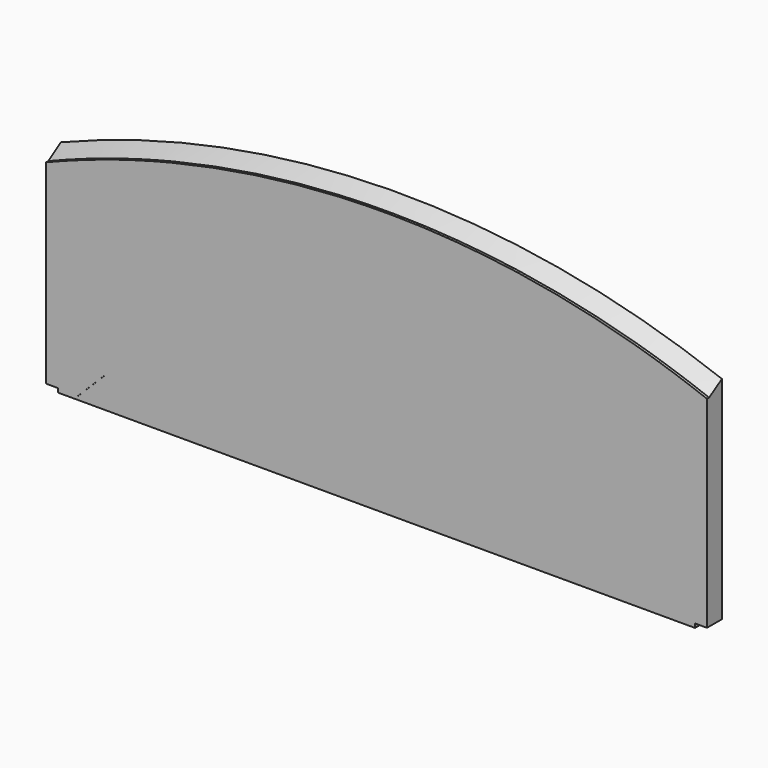
from build123d import *

# Parameters (mm, degrees)
F1_DEPTH    = 19.05
F2_T2_ANGLE = 47.80727079
F4_DEPTH    = 3.175


# Not quite as in the source:
# - a fillet or chamfer that OpenCascade refuses, or shapes differently, is made with other operations: its cross-section is extruded or revolved along the edge and cut away or added


with BuildPart() as f1:
    # F0 (on Front) → F1 (new body)
    with BuildSketch(Plane.XZ):
        with BuildLine():
            Line((-379.386894745, -118.26875), (379.4125, -118.26875))
            Line((379.4125, -118.26875), (379.4125, -113.50625))
            Line((379.4125, -113.50625), (393.7, -113.50625))
            Line((393.7, -113.50625), (393.7, 124.61875))
            ThreePointArc((393.7, 124.61875), (-0.5889314831, 196.0563533265), (-393.674394745, 118.26875))
            Line((-393.674394745, 118.26875), (-393.674394745, -113.50625))
            Line((-393.674394745, -113.50625), (-379.386894745, -113.50625))
            Line((-379.386894745, -113.50625), (-379.386894745, -118.26875))
        make_face()
        with BuildLine():
            ThreePointArc((-393.674394745, 118.26875), (-0.5889314831, 196.0563533265), (393.7, 124.61875))
            Line((393.7, 124.61875), (393.7, 138.90625))
            ThreePointArc((393.7, 138.90625), (-0.7824585401, 208.7544433839), (-393.7768174305, 130.96875))
            Line((-393.7768174305, 130.96875), (-393.674394745, 118.26875))
        make_face()
    extrude(amount=F1_DEPTH)

    # F2: chamfer of 19.558 x 11.43 on 1 edges, made by hand

    # F2_s1 → F2_t2 (revolve, cut)
    with BuildSketch(Plane(origin=(327.911656241, 0, -141.3984070605), x_dir=(0, 1, 0), z_dir=(0.9182658757, 0, -0.3959643691))):
        Polygon((0.508, 284.621375818), (-19.05, 273.191375818), (-19.05, 284.621375818), align=None)
    revolve(axis=Axis((10.1741912427, -19.05, -878.2512511865), (0, -1, 0)), revolution_arc=F2_T2_ANGLE, mode=Mode.SUBTRACT)

    # F3 (on face) → F4 (join)
    with BuildSketch(Plane.XZ.offset(19.05)):
        Polygon((71.1841804533, -118.26875), (178.9472539061, -118.26875), (218.205169263, -79.0108346431), (164.3236325366, -25.1292979167), (110.4420958102, -79.0108346431), align=None)
        Polygon((218.205169263, -79.0108346431), (178.9472539061, -118.26875), (257.4630846199, -118.26875), align=None)
        Polygon((393.7, -113.50625), (393.7, -38.9795184745), (379.8497794422, -25.1292979167), (325.9682427158, -79.0108346431), (286.710327359, -118.26875), (379.4125, -118.26875), (379.4125, -113.50625), align=None)
        Polygon((379.8497794422, -25.1292979167), (393.7, -38.9795184745), (393.7, -11.279077359), align=None)
        Polygon((218.205169263, -79.0108346431), (257.4630846199, -118.26875), (286.710327359, -118.26875), (325.9682427158, -79.0108346431), (272.0867059894, -25.1292979167), (218.205169263, 28.7522388097), (164.3236325366, -25.1292979167), align=None)
        Polygon((41.9369377142, -118.26875), (71.1841804533, -118.26875), (110.4420958102, -79.0108346431), (56.5605590837, -25.1292979167), (2.6790223573, 28.7522388097), (-51.2025143691, -25.1292979167), (2.6790223573, -79.0108346431), align=None)
        Polygon((-36.5788929995, -118.26875), (41.9369377142, -118.26875), (2.6790223573, -79.0108346431), align=None)
        Polygon((-144.3419664524, -118.26875), (-36.5788929995, -118.26875), (2.6790223573, -79.0108346431), (-51.2025143691, -25.1292979167), (-105.0840510955, -79.0108346431), align=None)
        Polygon((325.9682427158, -79.0108346431), (379.8497794422, -25.1292979167), (393.7, -11.279077359), (393.7, 68.7835549784), (379.8497794422, 82.6337755361), (325.9682427158, 28.7522388097), (272.0867059894, -25.1292979167), align=None)
        Polygon((110.4420958102, -79.0108346431), (164.3236325366, -25.1292979167), (218.205169263, 28.7522388097), (164.3236325366, 82.6337755361), (110.4420958102, 28.7522388097), (56.5605590837, -25.1292979167), align=None)
        Polygon((-173.5892091915, -118.26875), (-144.3419664524, -118.26875), (-105.0840510955, -79.0108346431), (-158.9655878219, -25.1292979167), (-212.8471245483, 28.7522388097), (-266.7286612747, -25.1292979167), (-212.8471245483, -79.0108346431), align=None)
        Polygon((379.8497794422, 82.6337755361), (393.7, 68.7835549784), (393.7, 96.4839960939), align=None)
        Polygon((218.205169263, 28.7522388097), (272.0867059894, -25.1292979167), (325.9682427158, 28.7522388097), (272.0867059894, 82.6337755361), (218.205169263, 136.5153122625), (164.3236325366, 82.6337755361), align=None)
        Polygon((2.6790223573, 28.7522388097), (56.5605590837, -25.1292979167), (110.4420958102, 28.7522388097), (56.5605590837, 82.6337755361), (2.6790223573, 136.5153122625), (-51.2025143691, 82.6337755361), align=None)
        Polygon((-105.0840510955, -79.0108346431), (-51.2025143691, -25.1292979167), (2.6790223573, 28.7522388097), (-51.2025143691, 82.6337755361), (-105.0840510955, 28.7522388097), (-158.9655878219, -25.1292979167), align=None)
        Polygon((-252.1050399052, -118.26875), (-173.5892091915, -118.26875), (-212.8471245483, -79.0108346431), align=None)
        Polygon((-359.868113358, -118.26875), (-252.1050399052, -118.26875), (-212.8471245483, -79.0108346431), (-266.7286612747, -25.1292979167), (-320.6101980012, -79.0108346431), align=None)
        with BuildLine():
            Line((325.9682427158, 28.7522388097), (379.8497794422, 82.6337755361))
            Line((379.8497794422, 82.6337755361), (393.7, 96.4839960939))
            Line((393.7, 96.4839960939), (393.7, 126.6814901711))
            ThreePointArc((393.7, 126.6814901711), (365.104665334, 137.1335129285), (336.2249713921, 146.7720409389))
            Line((336.2249713921, 146.7720409388), (325.9682427158, 136.5153122625))
            Line((325.9682427158, 136.5153122625), (272.0867059894, 82.6337755361))
            Line((272.0867059894, 82.6337755361), (325.9682427158, 28.7522388097))
        make_face()
        with BuildLine():
            Line((110.4420958102, 28.7522388097), (164.3236325366, 82.6337755361))
            Line((164.3236325366, 82.6337755361), (218.205169263, 136.5153122625))
            Line((218.205169263, 136.5153122625), (169.1544903585, 185.565991167))
            ThreePointArc((169.1544903585, 185.565991167), (164.9380697375, 186.1875692954), (160.7192193307, 186.792435783))
            Line((160.7192193307, 186.792435783), (110.4420958102, 136.5153122625))
            Line((110.4420958102, 136.5153122625), (56.5605590837, 82.6337755361))
            Line((56.5605590837, 82.6337755361), (110.4420958102, 28.7522388097))
        make_face()
        Polygon((-212.8471245483, 28.7522388097), (-158.9655878219, -25.1292979167), (-105.0840510955, 28.7522388097), (-158.9655878219, 82.6337755361), (-212.8471245483, 136.5153122625), (-266.7286612747, 82.6337755361), align=None)
        with BuildLine():
            Line((218.205169263, 136.5153122625), (272.0867059894, 82.6337755361))
            Line((272.0867059894, 82.6337755361), (325.9682427158, 136.5153122625))
            Line((325.9682427158, 136.5153122625), (306.8177631195, 155.6657918589))
            ThreePointArc((306.8177631195, 155.6657918589), (238.4761479453, 172.8719942997), (169.1544903585, 185.565991167))
            Line((169.1544903585, 185.565991167), (218.205169263, 136.5153122625))
        make_face()
        with BuildLine():
            Line((2.6790223573, 136.5153122625), (56.5605590838, 82.6337755361))
            Line((56.5605590837, 82.6337755361), (110.4420958102, 136.5153122625))
            Line((110.4420958102, 136.5153122625), (56.5605590837, 190.3968489889))
            Line((56.5605590837, 190.3968489889), (50.3274681554, 196.6299399173))
            ThreePointArc((50.3274681554, 196.6299399173), (2.3207372282, 197.350991232), (-45.670346508, 195.92901685))
            Line((-45.670346508, 195.92901685), (-51.2025143691, 190.3968489889))
            Line((-51.2025143691, 190.3968489889), (2.6790223573, 136.5153122625))
        make_face()
        Polygon((-105.0840510955, 28.7522388097), (-51.2025143691, 82.6337755361), (2.6790223573, 136.5153122625), (-51.2025143691, 190.3968489889), (-105.0840510955, 136.5153122625), (-158.9655878219, 82.6337755361), align=None)
        Polygon((-266.7286612747, -25.1292979167), (-212.8471245483, 28.7522388097), (-266.7286612747, 82.6337755361), (-320.6101980012, 28.7522388097), (-374.4917347276, -25.1292979167), (-320.6404889111, -78.9805437332), (-320.6101980012, -79.0108346431), align=None)
        Polygon((-379.386894745, -118.26875), (-359.9286951779, -118.26875), (-320.6404889111, -78.9805437332), (-374.4917347276, -25.1292979167), (-393.674394745, -5.9466378993), (-393.674394745, -113.50625), (-379.386894745, -113.50625), align=None)
        with BuildLine():
            Line((325.9682427158, 136.5153122625), (336.2249713921, 146.7720409388))
            ThreePointArc((336.2249713921, 146.7720409389), (321.5531223101, 151.3239145605), (306.8177631195, 155.6657918589))
            Line((306.8177631195, 155.6657918589), (325.9682427158, 136.5153122625))
        make_face()
        with BuildLine():
            Line((56.5605590837, 190.3968489889), (110.4420958102, 136.5153122625))
            Line((110.4420958102, 136.5153122625), (160.7192193307, 186.792435783))
            ThreePointArc((160.7192193307, 186.792435783), (111.6070850178, 192.5863782868), (62.2805468294, 196.1168367345))
            Line((62.2805468293, 196.1168367345), (56.5605590837, 190.3968489889))
        make_face()
        with BuildLine():
            Line((-320.6101980012, 28.7522388097), (-266.7286612747, 82.6337755361))
            Line((-266.7286612747, 82.6337755361), (-212.8471245483, 136.5153122625))
            Line((-212.8471245483, 136.5153122625), (-243.3958660177, 167.0640537319))
            ThreePointArc((-243.3958660177, 167.0640537319), (-275.7499582928, 158.6813605815), (-307.8279930641, 149.2975171996))
            Line((-307.8279930641, 149.2975171996), (-320.6101980012, 136.5153122625))
            Line((-320.6101980012, 136.5153122625), (-374.4917347276, 82.6337755361))
            Line((-374.4917347276, 82.6337755361), (-320.6101980012, 28.7522388097))
        make_face()
        with BuildLine():
            Line((-212.8471245483, 136.5153122625), (-158.9655878219, 82.6337755361))
            Line((-158.9655878219, 82.6337755361), (-105.0840510955, 136.5153122625))
            Line((-105.0840510955, 136.5153122625), (-153.4329816595, 184.8642428265))
            ThreePointArc((-153.4329816595, 184.8642428265), (-198.6042128715, 176.9233498209), (-243.3958660177, 167.0640537319))
            Line((-243.3958660177, 167.0640537319), (-212.8471245483, 136.5153122625))
        make_face()
        with BuildLine():
            Line((50.3274681554, 196.6299399173), (56.5605590837, 190.3968489889))
            Line((56.5605590837, 190.3968489889), (62.2805468293, 196.1168367345))
            ThreePointArc((62.2805468294, 196.1168367345), (56.3047208944, 196.3900074992), (50.3274681554, 196.6299399173))
        make_face()
        with BuildLine():
            Line((-105.0840510955, 136.5153122625), (-51.2025143691, 190.3968489889))
            Line((-51.2025143691, 190.3968489889), (-45.670346508, 195.92901685))
            ThreePointArc((-45.670346508, 195.92901685), (-99.6910472687, 191.75411796), (-153.4329816595, 184.8642428265))
            Line((-153.4329816595, 184.8642428265), (-105.0840510955, 136.5153122625))
        make_face()
        Polygon((-374.4917347276, -25.1292979167), (-320.6101980012, 28.7522388097), (-374.4917347276, 82.6337755361), (-393.674394745, 101.8164355535), (-393.674394745, -5.9466378993), align=None)
        with BuildLine():
            Line((-393.674394745, 101.8164355535), (-374.4917347276, 82.6337755361))
            Line((-374.4917347276, 82.6337755361), (-320.6101980012, 136.5153122625))
            Line((-320.6101980012, 136.5153122625), (-327.1969421676, 143.102056429))
            ThreePointArc((-327.1969421676, 143.102056429), (-360.6383542509, 131.4417302391), (-393.6777661416, 118.6867895926))
            Line((-393.6777661416, 118.6867895926), (-393.674394745, 118.26875))
            Line((-393.674394745, 118.26875), (-393.674394745, 101.8164355535))
        make_face()
        with BuildLine():
            Line((-320.6101980012, 136.5153122625), (-307.8279930641, 149.2975171996))
            ThreePointArc((-307.8279930641, 149.2975171996), (-317.5271092238, 146.2455610624), (-327.1969421676, 143.102056429))
            Line((-327.1969421676, 143.102056429), (-320.6101980012, 136.5153122625))
        make_face()
    extrude(amount=F4_DEPTH)


solid = f1.part
